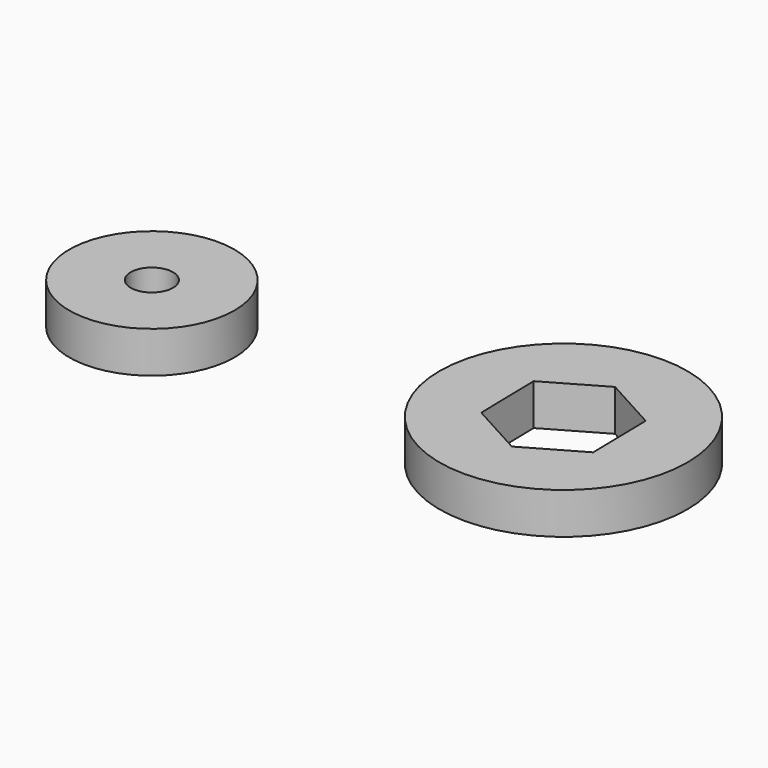
from build123d import *

# Parameters (mm, degrees)
F0_R     = 6.35
F0_R_2   = 1.6256
F1_DEPTH = 3.175
F0_R_3   = 9.525


# Not quite as in the source:
# - a length typed as a fraction of an inch, garbled in the dataset ("3 / 203.2 mm" for 3/8 in), is restored


with BuildPart() as f1:
    # F0 (on Top) → F1 (new body)
    with BuildSketch(Plane.XY):
        with Locations((-30.3984060884, -1.5536330175)):
            Circle(F0_R)
        with Locations((-30.3984060884, -1.5536330175)):
            Circle(F0_R_2, mode=Mode.SUBTRACT)
    extrude(amount=F1_DEPTH)


with BuildPart() as f1b:
    # F0 (on Top) → F1, piece 2 (new body)
    with BuildSketch(Plane.XY):
        Circle(F0_R_3)
        Polygon((-4.1838677777, -2.6657365395), (-4.2884325113, 2.4940423964), (0, 4.9609375), (4.1838677777, 2.6657365395), (4.2884325113, -2.4940423964), (0, -4.9609375), align=None, mode=Mode.SUBTRACT)
    extrude(amount=F1_DEPTH)


solid = Compound([f1.part, f1b.part])
